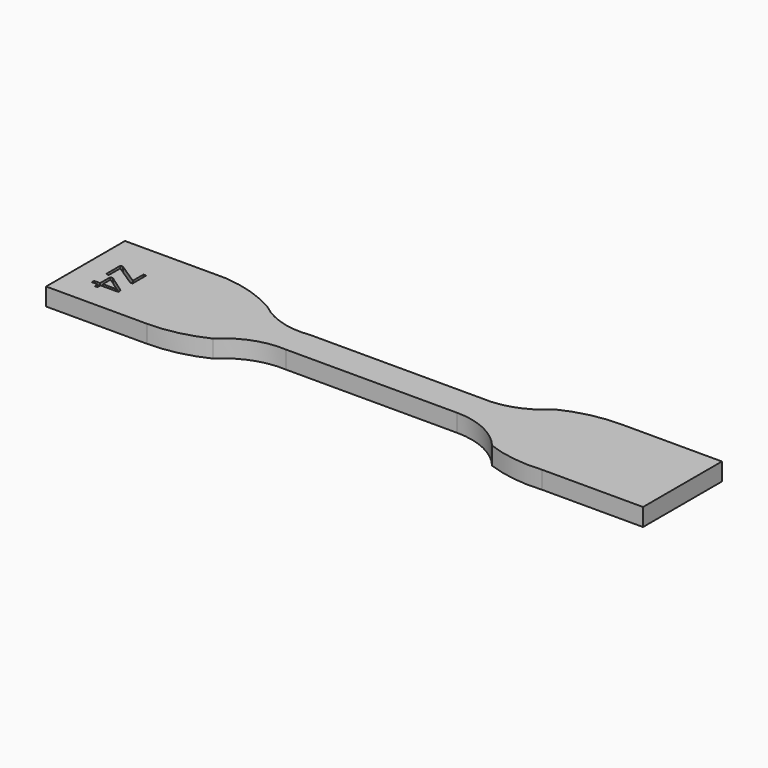
from build123d import *

# Parameters (mm, degrees)
F1_DEPTH     = 3.4
F2_TEXT_SIZE = 7.0564552314
F3_DEPTH     = 1


# Not quite as in the source:
# - Text() gives the source's letters only with a copy of the font that has no kerning and outlines rounded to 1/6400 em; it was checked with that copy


with BuildPart() as f1:
    # F0 (on Top) → F1 (new body)
    with BuildSketch(Plane.XY):
        with BuildLine():
            Line((-14.4320548165, 19.7811394548), (-33.8720548165, 19.7811394548))
            Line((-33.8720548165, 19.7811394548), (-33.8720548165, 0.7811394548))
            Line((-33.8720548165, 0.7811394548), (-14.4320548165, 0.7811394548))
            ThreePointArc((-14.4320548165, 0.7811394548), (-8.9053122052, 1.3996892086), (-3.6520548165, 3.2247301661))
            ThreePointArc((-3.6520548165, 3.2247301661), (1.3014698263, 6.4128780055), (7.1279451835, 7.2811394548))
            Line((7.1279451835, 7.2811394548), (40.1279451835, 7.2811394548))
            ThreePointArc((40.1279451835, 7.2811394548), (46.0837574042, 5.9511158081), (50.9079451835, 2.2137538538))
            ThreePointArc((50.9079451835, 2.2137538538), (56.2191047011, 0.9041953221), (61.6879451835, 0.7811394548))
            Line((61.6879451835, 0.7811394548), (81.1279451835, 0.7811394548))
            Line((81.1279451835, 0.7811394548), (81.1279451835, 19.7811394548))
            Line((81.1279451835, 19.7811394548), (61.6879451835, 19.7811394548))
            ThreePointArc((61.6879451835, 19.7811394548), (56.1612025723, 19.162589701), (50.9079451835, 17.3375487435))
            ThreePointArc((50.9079451835, 17.3375487435), (45.9544205407, 14.1494009041), (40.1279451835, 13.2811394548))
            Line((40.1279451835, 13.2811394548), (7.1279451835, 13.2811394548))
            ThreePointArc((7.1279451835, 13.2811394548), (1.4167452884, 13.6925537245), (-3.6520548165, 16.3560723447))
            ThreePointArc((-3.6520548165, 16.3560723447), (-8.8458057958, 18.686276846), (-14.4320548165, 19.7811394548))
        make_face()
    extrude(amount=F1_DEPTH)

    # F2 (on face) → F3 (cut)
    with BuildSketch(Plane.XY.offset(3.4)):
        with Locations(Location((-29.3720550835, 13.353464842), (0, 0, -90))):
            Text('Z4', F2_TEXT_SIZE, font='Open Sans', text_align=(TextAlign.LEFT, TextAlign.BOTTOM))
    extrude(amount=-F3_DEPTH, mode=Mode.SUBTRACT)


solid = f1.part
